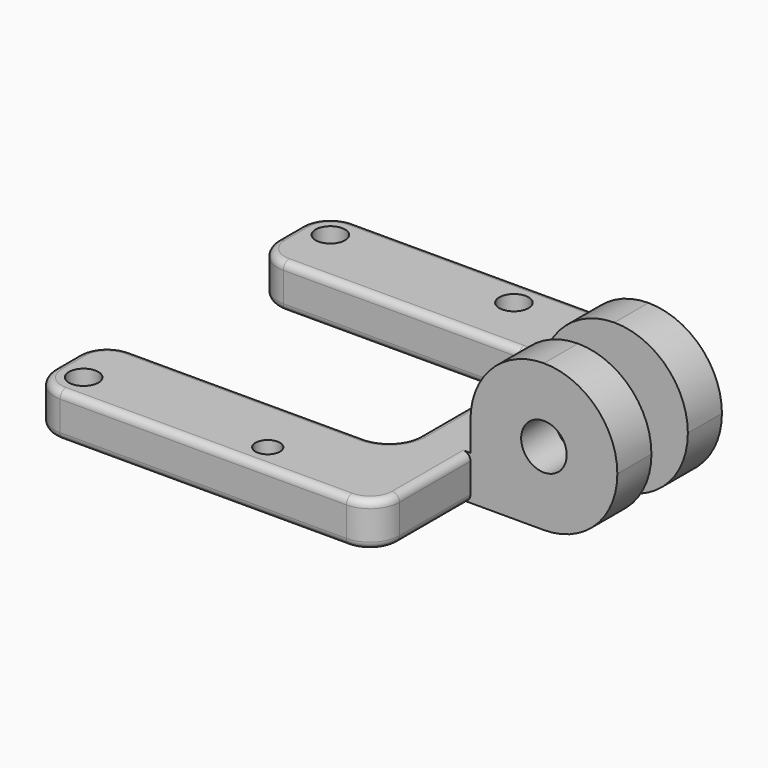
from build123d import *

# Parameters (mm, degrees)
F0_R     = 1
F0_R_2   = 0.8289430236
F1_DEPTH = 3
F0_W     = 10
F0_H     = 2.9
F2_DEPTH = 10
F3_R     = 4.99999
F5_R     = 0.5
F4_R     = 1.55
F6_DEPTH = 8.9


# Not quite as in the source:
# - a fillet or chamfer is up to 0.001 mm smaller than in the source, because OpenCascade refuses the exact size


with BuildPart() as f1:
    # F0 (on Top) → F1 (new body)
    with BuildSketch(Plane.XY):
        with BuildLine():
            ThreePointArc((11.75, 10.5), (11.1642135624, 11.9142135624), (9.75, 12.5))
            Line((9.75, 12.5), (-9.75, 12.5))
            ThreePointArc((-9.75, 12.5), (-11.1642135624, 11.9142135624), (-11.75, 10.5))
            Line((-11.75, 10.5), (-11.75, 8.5))
            ThreePointArc((-11.75, 8.5), (-11.1642135624, 7.0857864376), (-9.75, 6.5))
            Line((-9.75, 6.5), (6.25, 6.5))
            ThreePointArc((6.25, 6.5), (7.6642135624, 5.9142135624), (8.25, 4.5))
            Line((8.25, 4.5), (8.25, -4.5))
            ThreePointArc((8.25, -4.5), (7.6642135624, -5.9142135624), (6.25, -6.5))
            Line((6.25, -6.5), (-9.75, -6.5))
            ThreePointArc((-9.75, -6.5), (-11.1642135624, -7.0857864376), (-11.75, -8.5))
            Line((-11.75, -8.5), (-11.75, -10.5))
            ThreePointArc((-11.75, -10.5), (-11.1642135624, -11.9142135624), (-9.75, -12.5))
            Line((-9.75, -12.5), (9.75, -12.5))
            ThreePointArc((9.75, -12.5), (11.1642135624, -11.9142135624), (11.75, -10.5))
            Line((11.75, -10.5), (11.75, -4.45))
            Line((11.75, -4.45), (11.75, -1.55))
            Line((11.75, -1.55), (11.75, 1.55))
            Line((11.75, 1.55), (11.75, 4.45))
            Line((11.75, 4.45), (11.75, 10.5))
        make_face()
        with Locations((-9.75, -10.5)):
            Circle(F0_R, mode=Mode.SUBTRACT)
        with Locations((2.9210569764, -10.6710569764)):
            Circle(F0_R_2, mode=Mode.SUBTRACT)
        with Locations((-9.75, 10.5)):
            Circle(F0_R, mode=Mode.SUBTRACT)
        with Locations((2.75, 10.5)):
            Circle(F0_R, mode=Mode.SUBTRACT)
    extrude(amount=F1_DEPTH)

    # F0 (on Top) → F2 (join)
    with BuildSketch(Plane.XY):
        with Locations((16.75, 3)):
            Rectangle(F0_W, F0_H)
        with Locations((16.75, -3)):
            Rectangle(F0_W, F0_H)
    extrude(amount=F2_DEPTH)

    # F3 (radius 5 in the source; OpenCascade refuses exactly that, so slightly less here)
    f3_edges = [f1.edges().sort_by_distance(p)[0] for p in [
        (11.75, -3, 10),
        (11.75, 3, 10),
        (21.75, 3, 10),
        (21.75, -3, 10),
        (21.75, 3, 0),
        (21.75, -3, 0),
    ]]
    fillet(f3_edges, radius=F3_R)

    # F5
    f5_edges = [f1.edges().sort_by_distance(p)[0] for p in [
        (-1.75, 6.5, 3),
        (11.75, 7.475, 3),
        (11.75, 0, 3),
        (11.75, -7.475, 3),
        (0, -12.5, 0),
        (11.75, 0, 0),
    ]]
    fillet(f5_edges, radius=F5_R)

    # F4 (on face) → F6 (cut)
    with BuildSketch(Plane.XZ.offset(4.45)):
        with Locations((16.75, 5)):
            Circle(F4_R)
    extrude(amount=-F6_DEPTH, mode=Mode.SUBTRACT)


solid = f1.part
